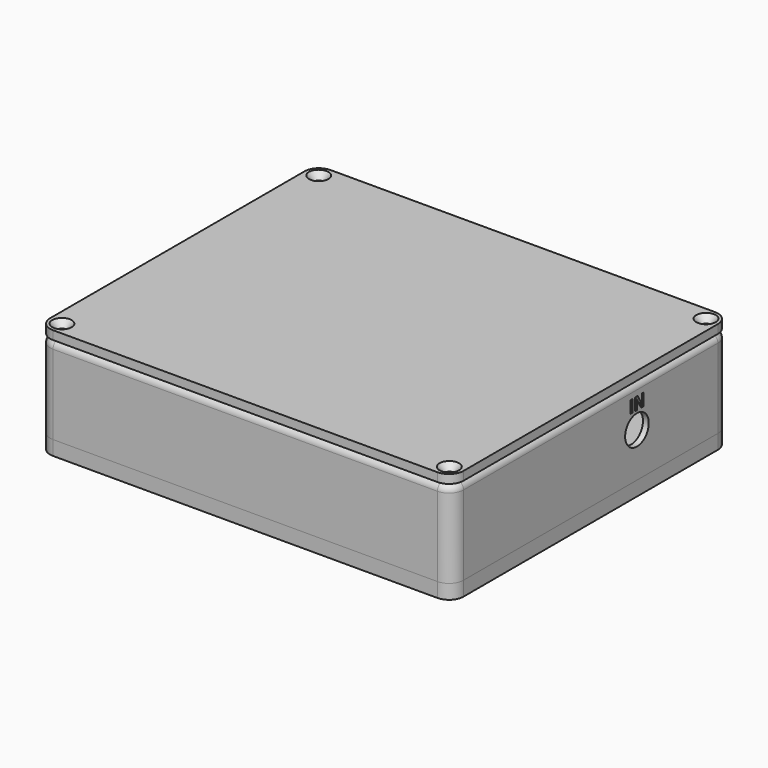
from build123d import *

# Parameters (mm, degrees)
F0_W           = 143
F0_H           = 120
F0_R           = 6
F0_R_2         = 2.5
F0_R_3         = 3.6
F1_DEPTH       = 30
F2_R           = 6
F2_R_2         = 3.6
F2_R_3         = 2.5
F3_DEPTH       = 25
F2_R_4         = 1.4
F4_DEPTH       = 10
F5_W           = 143
F5_H           = 3
F6_DEPTH       = 120
F7_R           = 5
F7_2_R         = 5
F9_D           = 2.5
F9_DEPTH       = 13.5
F9_CSINK_D     = 6.72
F9_CSINK_ANGLE = 90
F9_TIP         = 0.7510757738
F10_R          = 5.1
F11_DEPTH      = 158.2
F12_R          = 6.1
F13_DEPTH      = 25
F14_TEXT_SIZE  = 5.9218834698
F15_DEPTH      = 1.4
F16_TEXT_SIZE  = 6.3812062662
F17_DEPTH      = 1.5
F18_R          = 2.5
F21_DEPTH      = 3
F23_DEPTH      = 2


# Not quite as in the source:
# - Text() gives the source's letters only with a copy of the font that has no kerning and outlines rounded to 1/6400 em; it was checked with that copy


with BuildPart() as f1:
    # F0 (on Top) → F1 (new body)
    with BuildSketch(Plane.XY):
        Rectangle(F0_W, F0_H)
        with Locations((-51.5, -33)):
            Circle(F0_R, mode=Mode.SUBTRACT)
        with Locations((-36.5, -33)):
            Circle(F0_R_2, mode=Mode.SUBTRACT)
        with Locations((0, -33)):
            Circle(F0_R, mode=Mode.SUBTRACT)
        with Locations((36.5, -33)):
            Circle(F0_R_2, mode=Mode.SUBTRACT)
        with Locations((51.5, -33)):
            Circle(F0_R, mode=Mode.SUBTRACT)
        with Locations((0, -18)):
            Circle(F0_R_2, mode=Mode.SUBTRACT)
        with Locations((-35, 24)):
            Circle(F0_R_3, mode=Mode.SUBTRACT)
        with Locations((-51, 45)):
            Circle(F0_R, mode=Mode.SUBTRACT)
        with Locations((-19, 45)):
            Circle(F0_R, mode=Mode.SUBTRACT)
        Circle(F0_R_3, mode=Mode.SUBTRACT)
        with Locations((0, 24)):
            Circle(F0_R_3, mode=Mode.SUBTRACT)
        with Locations((35.75, 0)):
            Circle(F0_R_3, mode=Mode.SUBTRACT)
        with Locations((35.75, 24)):
            Circle(F0_R_3, mode=Mode.SUBTRACT)
        with Locations((35.75, 45)):
            Circle(F0_R_3, mode=Mode.SUBTRACT)
    extrude(amount=-F1_DEPTH)

    # F2 (on face) → F3 (cut)
    with BuildSketch(Plane(origin=(0, 0, -30), x_dir=(1, 0, 0), z_dir=(0, 0, -1))):
        with BuildLine():
            Line((-69.5, 50.2020410289), (-69.5, -50.2020410289))
            ThreePointArc((-69.5, -50.2020410289), (-64.4289321881, -52.9289321881), (-61.7020410289, -58))
            Line((-61.7020410289, -58), (61.7020410289, -58))
            ThreePointArc((61.7020410289, -58), (64.4289321881, -52.9289321881), (69.5, -50.2020410289))
            Line((69.5, -50.2020410289), (69.5, 50.2020410289))
            ThreePointArc((69.5, 50.2020410289), (64.4289321881, 52.9289321881), (61.7020410289, 58))
            Line((61.7020410289, 58), (-61.7020410289, 58))
            ThreePointArc((-61.7020410289, 58), (-64.4289321881, 52.9289321881), (-69.5, 50.2020410289))
        make_face()
        with Locations((-51, -45)):
            Circle(F2_R, mode=Mode.SUBTRACT)
        with Locations((-19, -45)):
            Circle(F2_R, mode=Mode.SUBTRACT)
        with Locations((-35, -24)):
            Circle(F2_R_2, mode=Mode.SUBTRACT)
        with Locations((35.75, -45)):
            Circle(F2_R_2, mode=Mode.SUBTRACT)
        with Locations((0, -24)):
            Circle(F2_R_2, mode=Mode.SUBTRACT)
        with Locations((35.75, -24)):
            Circle(F2_R_2, mode=Mode.SUBTRACT)
        with Locations((-51.5, 33)):
            Circle(F2_R, mode=Mode.SUBTRACT)
        with Locations((-36.5, 33)):
            Circle(F2_R_3, mode=Mode.SUBTRACT)
        Circle(F2_R_2, mode=Mode.SUBTRACT)
        with Locations((0, 18)):
            Circle(F2_R_3, mode=Mode.SUBTRACT)
        with Locations((35.75, 0)):
            Circle(F2_R_2, mode=Mode.SUBTRACT)
        with Locations((0, 33)):
            Circle(F2_R, mode=Mode.SUBTRACT)
        with Locations((36.5, 33)):
            Circle(F2_R_3, mode=Mode.SUBTRACT)
        with Locations((51.5, 33)):
            Circle(F2_R, mode=Mode.SUBTRACT)
    extrude(amount=-F3_DEPTH, mode=Mode.SUBTRACT)

    # F2 (on face) → F4 (cut)
    with BuildSketch(Plane(origin=(0, 0, -30), x_dir=(1, 0, 0), z_dir=(0, 0, -1))):
        with Locations((-67, -55.5)):
            Circle(F2_R_4)
        with Locations((-67, 55.5)):
            Circle(F2_R_4)
        with Locations((67, 55.5)):
            Circle(F2_R_4)
        with Locations((67, -55.5)):
            Circle(F2_R_4)
    extrude(amount=-F4_DEPTH, mode=Mode.SUBTRACT)

    # F7
    f7_edges = [f1.edges().sort_by_distance(p)[0] for p in [
        (-71.5, -60, -15),
        (71.5, -60, -15),
        (71.5, 60, -15),
        (-71.5, 60, -15),
    ]]
    fillet(f7_edges, radius=F7_R)

    # F10 (on face) → F11 (cut)
    with BuildSketch(Plane(origin=(-71.5, 0, 0), x_dir=(0, -1, 0), z_dir=(-1, 0, 0))):
        with Locations((-20, -14.7)):
            Circle(F10_R)
    extrude(amount=-F11_DEPTH, mode=Mode.SUBTRACT)

    # F12 (on face) → F13 (cut)
    with BuildSketch(Plane(origin=(0, 60, 0), x_dir=(-1, 0, 0), z_dir=(0, 1, 0))):
        with Locations((0, -15)):
            Circle(F12_R)
    extrude(amount=-F13_DEPTH, mode=Mode.SUBTRACT)

    # F14 (on face) → F15 (cut)
    with BuildSketch(Plane.YZ.offset(71.5)):
        with Locations((16.6865211398, -8.7)):
            Text('IN', F14_TEXT_SIZE, font='Open Sans', font_style=FontStyle.BOLD, text_align=(TextAlign.LEFT, TextAlign.BOTTOM))
    extrude(amount=-F15_DEPTH, mode=Mode.SUBTRACT)

    # F16 (on face) → F17 (cut)
    with BuildSketch(Plane(origin=(-71.5, 0, 0), x_dir=(0, -1, 0), z_dir=(-1, 0, 0))):
        with Locations((-26.9420544732, -8.7)):
            Text('OUT', F16_TEXT_SIZE, font='Open Sans', font_style=FontStyle.BOLD, text_align=(TextAlign.LEFT, TextAlign.BOTTOM))
    extrude(amount=-F17_DEPTH, mode=Mode.SUBTRACT)

    # F18
    f18_edges = [f1.edges().sort_by_distance(p)[0] for p in [
        (0, -60, 0),
    ]]
    fillet(f18_edges, radius=F18_R)


with BuildPart() as f6:
    # F5 (on face) → F6 (new body, through all)
    with BuildSketch(Plane.XZ.offset(60)):
        with Locations((0, 1.8)):
            Rectangle(F5_W, F5_H)
    extrude(amount=-F6_DEPTH)

    # F7#2
    f7_2_edges = [f6.edges().sort_by_distance(p)[0] for p in [
        (-71.5, -60, 1.8),
        (71.5, -60, 1.8),
        (71.5, 60, 1.8),
        (-71.5, 60, 1.8),
    ]]
    fillet(f7_2_edges, radius=F7_2_R)

    # F9
    with Locations(Plane.XY.offset(3.3)):
        with Locations((-67, 55.5), (67, 55.5), (67, -55.5), (-67, -55.5)):
            CounterSinkHole(F9_D / 2, F9_CSINK_D / 2, depth=F9_DEPTH, counter_sink_angle=F9_CSINK_ANGLE)
            with Locations((0, 0, -(F9_DEPTH + F9_TIP / 2))):  # 118° drill point
                Cone(0, F9_D / 2, F9_TIP, mode=Mode.SUBTRACT)


with BuildPart() as f21:
    # F20 (on face) → F21 (new body)
    with BuildSketch(Plane(origin=(0, 0, -30), x_dir=(1, 0, 0), z_dir=(0, 0, -1))):
        with BuildLine():
            Line((-71.5, 55), (-71.5, -55))
            ThreePointArc((-71.5, -55), (-70.0355339059, -58.5355339059), (-66.5, -60))
            Line((-66.5, -60), (66.5, -60))
            ThreePointArc((66.5, -60), (70.0355339059, -58.5355339059), (71.5, -55))
            Line((71.5, -55), (71.5, 55))
            ThreePointArc((71.5, 55), (70.0355339059, 58.5355339059), (66.5, 60))
            Line((66.5, 60), (-66.5, 60))
            ThreePointArc((-66.5, 60), (-70.0355339059, 58.5355339059), (-71.5, 55))
        make_face()
        with BuildLine():
            ThreePointArc((-61.7020410289, -58), (-64.4289321881, -52.9289321881), (-69.5, -50.2020410289))
            Line((-69.5, -50.2020410289), (-69.5, 50.2020410289))
            ThreePointArc((-69.5, 50.2020410289), (-64.4289321881, 52.9289321881), (-61.7020410289, 58))
            Line((-61.7020410289, 58), (61.7020410289, 58))
            ThreePointArc((61.7020410289, 58), (64.4289321881, 52.9289321881), (69.5, 50.2020410289))
            Line((69.5, 50.2020410289), (69.5, -50.2020410289))
            ThreePointArc((69.5, -50.2020410289), (64.4289321881, -52.9289321881), (61.7020410289, -58))
            Line((61.7020410289, -58), (-61.7020410289, -58))
        make_face(mode=Mode.SUBTRACT)
    extrude(amount=F21_DEPTH)

    # F22 (on face) → F23 (join)
    with BuildSketch(Plane(origin=(0, 0, -33), x_dir=(1, 0, 0), z_dir=(0, 0, -1))):
        with BuildLine():
            Line((-71.5, 55), (-71.5, -55))
            ThreePointArc((-71.5, -55), (-70.0355339059, -58.5355339059), (-66.5, -60))
            Line((-66.5, -60), (66.5, -60))
            ThreePointArc((66.5, -60), (70.0355339059, -58.5355339059), (71.5, -55))
            Line((71.5, -55), (71.5, 55))
            ThreePointArc((71.5, 55), (70.0355339059, 58.5355339059), (66.5, 60))
            Line((66.5, 60), (-66.5, 60))
            ThreePointArc((-66.5, 60), (-70.0355339059, 58.5355339059), (-71.5, 55))
        make_face()
    extrude(amount=F23_DEPTH)


solid = Compound([f1.part, f6.part, f21.part])
